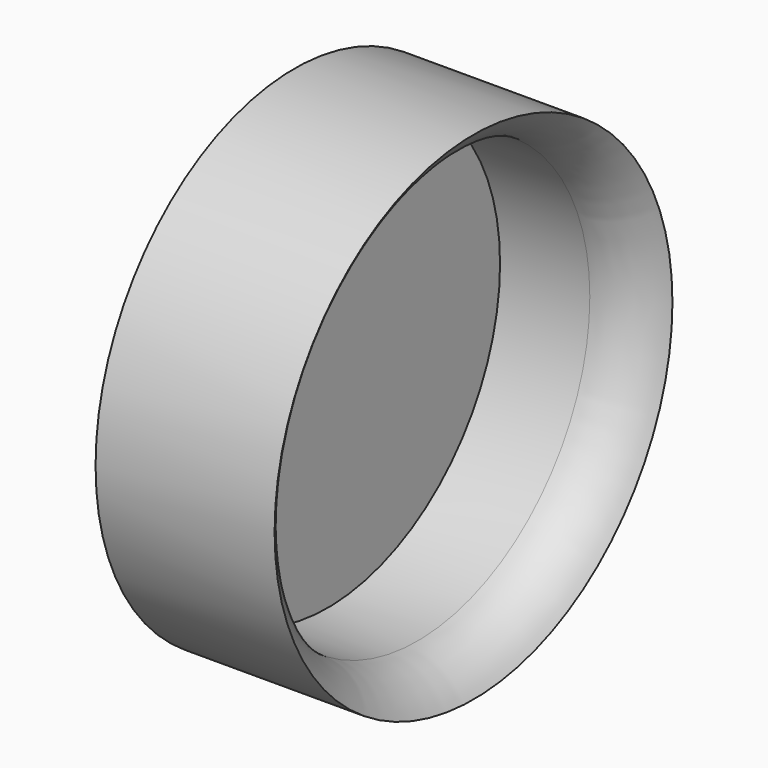
from build123d import *

# Parameters (mm, degrees)
F0_R     = 19.05
F0_R_2   = 12.7
F0_R_3   = 6.35
F1_DEPTH = 6.858
F2_T     = -2.54


# Not quite as in the source:
# - a fillet or chamfer that OpenCascade refuses, or shapes differently, is made with other operations: its cross-section is extruded or revolved along the edge and cut away or added
# - the program builds the solid bodies; features that only make, move or delete a surface that nothing else refers to are left out


with BuildPart() as f1:
    # F0 (on Right) → F1 (new body, symmetric)
    with BuildSketch(Plane.YZ):
        Circle(F0_R)
        Circle(F0_R_2, mode=Mode.SUBTRACT)
        Circle(F0_R_2)
        Circle(F0_R_3, mode=Mode.SUBTRACT)
        Circle(F0_R_3)
    extrude(amount=F1_DEPTH, both=True)

    # F2
    f2_openings = [f1.faces().sort_by_distance(p)[0] for p in [
        (6.858, 0, 0),
    ]]
    offset(amount=F2_T, openings=f2_openings)

    # F4: fillet of radius 4.9056819587 on 1 edges, made by hand

    # F4_s1 → F4_t2 (revolve, cut)
    with BuildSketch(Plane.XY):
        with BuildLine():
            ThreePointArc((6.858, 19.05), (5.0564518797, 17.1924723508), (2.5604117984, 16.51))
            Line((2.5604117984, 16.51), (6.858, 16.51))
            Line((6.858, 16.51), (6.858, 19.05))
        make_face()
    revolve(axis=Axis((6.858, 0, 0), (1, 0, 0)), mode=Mode.SUBTRACT)


solid = f1.part
